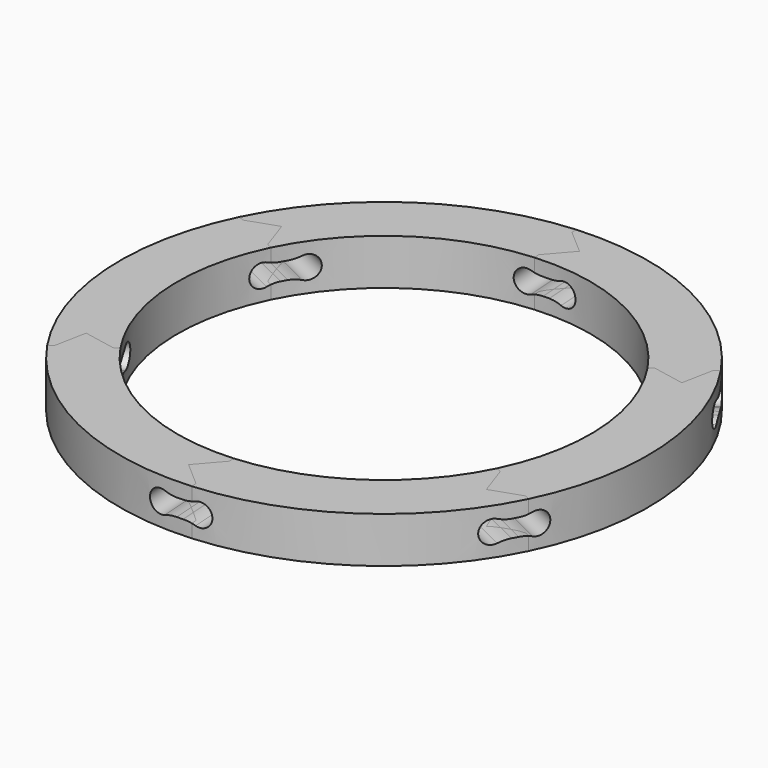
from build123d import *

# Parameters (mm, degrees)
F0_W          = 254
F0_H          = 203.2
F1_ANGLE_BACK = 34
F1_ANGLE      = 60
F3_DEPTH      = 203.2
F5_DEPTH      = 203.2
F9_DEPTH      = 254
F11_DEPTH     = 254
F13_DEPTH     = 76.2
F14_COUNT     = 6


with BuildPart() as f1:
    # F0 (on Front) → F1 (revolve)
    with BuildSketch(Plane.XZ, mode=Mode.PRIVATE) as f1_sk:
        with Locations((-1041.4, 0)):
            Rectangle(F0_W, F0_H)
    revolve(f1_sk.sketch.rotate(Axis((0, 0, 0), (0, 0, -1)), -F1_ANGLE_BACK), axis=Axis((0, 0, 0), (0, 0, -1)), revolution_arc=F1_ANGLE)

    # F2 (on face) → F3 (join, through all)
    with BuildSketch(Plane.XY.offset(101.6)):
        Polygon((-891.4656113022, 547.8371873701), (-1027.3215949199, 501.0582207799), (-844.686644712, 411.9812037524), align=None)
    extrude(amount=-F3_DEPTH)

    # F4 (on face) → F5 (cut, through all)
    with BuildSketch(Plane.XY.offset(101.6)):
        Polygon((-920.1737270514, -498.1132723028), (-947.5899454304, -639.1574886671), (-779.1295106872, -525.5294906818), align=None)
    extrude(amount=-F5_DEPTH, mode=Mode.SUBTRACT)

    # F8 (on face) → F9 (cut, symmetric)
    with BuildSketch(Plane(origin=(-936.004119816, 456.5197122661, 0), x_dir=(0.4383711468, 0.8987940463, 0), z_dir=(0.8987940463, -0.4383711468, 0))):
        with BuildLine():
            ThreePointArc((37.1095657574, 38.1), (10.1687973942, 40.50015), (-15.9233897985, 47.625))
            ThreePointArc((-15.9233897985, 47.625), (-84.4010416505, 0), (-15.9233897985, -47.625))
            ThreePointArc((-15.9233897985, -47.625), (10.1687973942, -40.50015), (37.1095657574, -38.1))
            Line((37.1095657574, -38.1), (64.4904342426, -38.1))
            ThreePointArc((64.4904342426, -38.1), (91.4312026058, -40.50015), (117.5233897985, -47.625))
            ThreePointArc((117.5233897985, -47.625), (186.0010416505, 0), (117.5233897985, 47.625))
            ThreePointArc((117.5233897985, 47.625), (91.4312026058, 40.50015), (64.4904342426, 38.1))
            Line((64.4904342426, 38.1), (37.1095657574, 38.1))
        make_face()
    extrude(amount=F9_DEPTH, both=True, mode=Mode.SUBTRACT)

    # F10 (on face) → F11 (cut, symmetric)
    with BuildSketch(Plane(origin=(-863.3597280588, -582.3434896744, 0), x_dir=(0.5591929035, -0.8290375726, 0), z_dir=(-0.8290375726, -0.5591929035, 0))):
        with BuildLine():
            ThreePointArc((-64.4904342426, 38.1), (-91.4312026058, 40.50015), (-117.5233897985, 47.625))
            ThreePointArc((-117.5233897985, 47.625), (-186.0010416505, 0), (-117.5233897985, -47.625))
            ThreePointArc((-117.5233897985, -47.625), (-91.4312026058, -40.50015), (-64.4904342426, -38.1))
            Line((-64.4904342426, -38.1), (-37.1095657574, -38.1))
            ThreePointArc((-37.1095657574, -38.1), (-10.1687973942, -40.50015), (15.9233897985, -47.625))
            ThreePointArc((15.9233897985, -47.625), (84.4010416505, 0), (15.9233897985, 47.625))
            ThreePointArc((15.9233897985, 47.625), (-10.1687973942, 40.50015), (-37.1095657574, 38.1))
            Line((-37.1095657574, 38.1), (-64.4904342426, 38.1))
        make_face()
    extrude(amount=F11_DEPTH, both=True, mode=Mode.SUBTRACT)

    # F12 (on face) → F13 (cut)
    with BuildSketch(Plane(origin=(0, 0, -101.6), x_dir=(1, 0, 0), z_dir=(0, 0, -1))):
        with BuildLine():
            ThreePointArc((-965.2, 25.4), (-972.6394877579, 43.3605122421), (-990.6, 50.8))
            Line((-990.6, 50.8), (-1092.2, 50.8))
            ThreePointArc((-1092.2, 50.8), (-1110.1605122421, 43.3605122421), (-1117.6, 25.4))
            Line((-1117.6, 25.4), (-1117.6, -25.4))
            ThreePointArc((-1117.6, -25.4), (-1110.1605122421, -43.3605122421), (-1092.2, -50.8))
            Line((-1092.2, -50.8), (-990.6, -50.8))
            ThreePointArc((-990.6, -50.8), (-972.6394877579, -43.3605122421), (-965.2, -25.4))
            Line((-965.2, -25.4), (-965.2, 25.4))
        make_face()
    extrude(amount=-F13_DEPTH, mode=Mode.SUBTRACT)


with BuildPart() as f14_1:
    # F14: instance of F1
    add(f1.part.rotate(Axis((0, 0, 0), (0, 0, -1)), 1 * 360 / F14_COUNT))


with BuildPart() as f14_2:
    # F14: instance of F1
    add(f1.part.rotate(Axis((0, 0, 0), (0, 0, -1)), 2 * 360 / F14_COUNT))


with BuildPart() as f14_3:
    # F14: instance of F1
    add(f1.part.rotate(Axis((0, 0, 0), (0, 0, -1)), 3 * 360 / F14_COUNT))


with BuildPart() as f14_4:
    # F14: instance of F1
    add(f1.part.rotate(Axis((0, 0, 0), (0, 0, -1)), 4 * 360 / F14_COUNT))


with BuildPart() as f14_5:
    # F14: instance of F1
    add(f1.part.rotate(Axis((0, 0, 0), (0, 0, -1)), 5 * 360 / F14_COUNT))


solid = Compound([f1.part, f14_1.part, f14_2.part, f14_3.part, f14_4.part, f14_5.part])
